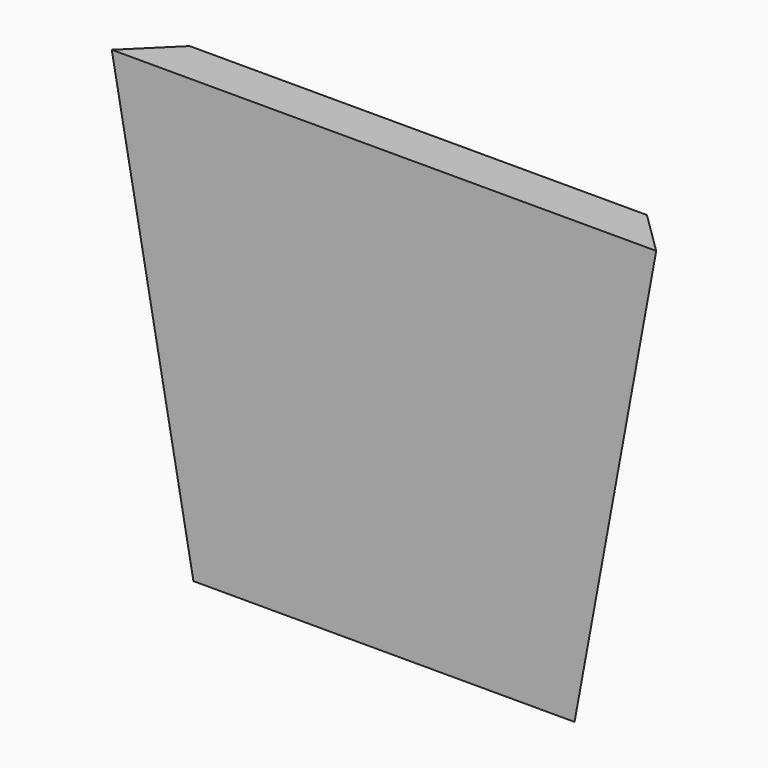
from build123d import *

# Parameters (mm, degrees)
F1_DEPTH = 20
F2_SIZE  = 19.99999
F3_SIZE  = 19.99999


# Not quite as in the source:
# - a fillet or chamfer is up to 0.001 mm smaller than in the source, because OpenCascade refuses the exact size


with BuildPart() as f1:
    # F0 (on Front) → F1 (new body)
    with BuildSketch(Plane.XZ):
        Polygon((-106.2891499103, -110.869043763), (71.5108500897, -110.869043763), (109.6108500897, 94.9895840839), (-144.3891499103, 94.9895840839), align=None)
    extrude(amount=F1_DEPTH)

    # F2 (size 20 in the source; OpenCascade refuses exactly that, so slightly less here)
    f2_edges = [f1.edges().sort_by_distance(p)[0] for p in [
        (90.56085, 0, -7.93973),
    ]]
    chamfer(f2_edges, length=F2_SIZE)

    # F3 (size 20 in the source; OpenCascade refuses exactly that, so slightly less here)
    f3_edges = [f1.edges().sort_by_distance(p)[0] for p in [
        (-125.33915, 0, -7.93973),
    ]]
    chamfer(f3_edges, length=F3_SIZE)


solid = f1.part
